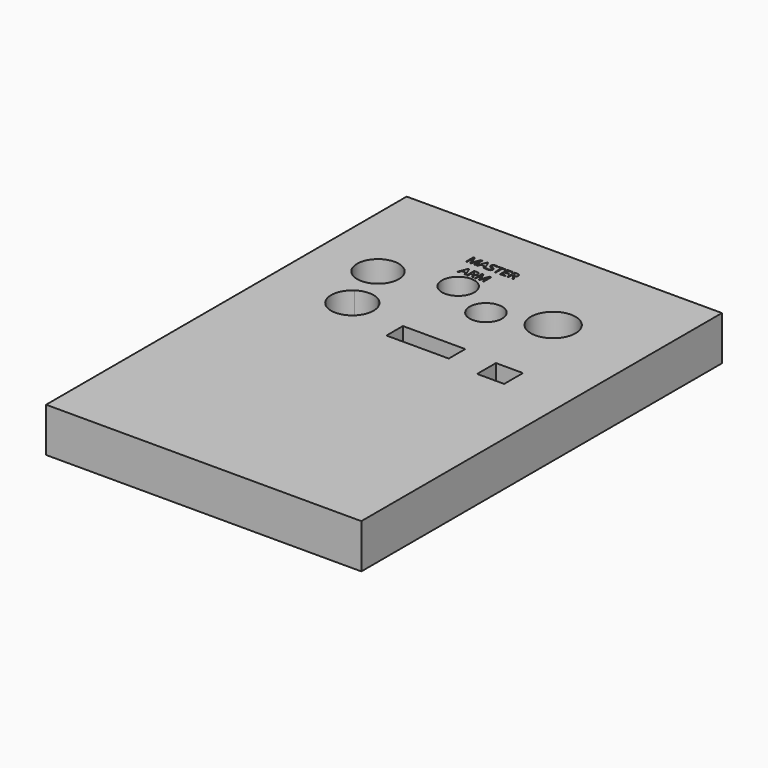
from build123d import *

# Parameters (mm, degrees)
F0_W     = 178
F0_H     = 254.5
F0_R     = 11.7739294938
F0_R_2   = 9.1574293731
F0_W_2   = 35.1873915642
F0_H_2   = 11.6184782237
F0_R_3   = 9.1574274825
F0_W_3   = 15.2700021863
F0_H_3   = 13.2782608271
F0_R_4   = 12.6405317235
F1_DEPTH = 25
F2_DEPTH = 25


with BuildPart() as f1:
    # F0 (on Top) → F1 (new body)
    with BuildSketch(Plane.XY):
        Rectangle(F0_W, F0_H)
        with Locations((-54.2288012803, 63.5412633419)):
            Circle(F0_R, mode=Mode.SUBTRACT)
        with BuildLine():
            ThreePointArc((-32.2966329035, 33.0012664199), (-49.9168302008, 22.4429384628), (-50.9175227463, 42.9599620402))
            ThreePointArc((-50.9175227463, 42.9599620402), (-44.2700982094, 44.9747317258), (-37.6226736725, 42.9599620402))
            ThreePointArc((-37.6226736725, 42.9599620402), (-33.7117702523, 38.6479984113), (-32.2966329035, 33.0012664199))
        make_face(mode=Mode.SUBTRACT)
        Polygon((-22.1080133536, 85.1738999287), (-22.7346302224, 85.1738999287), (-23.3828938556, 86.8293077656), (-25.4689583768, 86.8293077656), (-26.1092468863, 85.1738999287), (-26.7221921143, 85.1738999287), (-24.6646101781, 90.4010239174), (-24.1553415593, 90.4010239174), align=None, mode=Mode.SUBTRACT)
        with Locations((-17.7135802805, 74.4958370924)):
            Circle(F0_R_2, mode=Mode.SUBTRACT)
        with BuildLine():
            Line((-19.7006652743, 87.3385763844), (-20.7875607157, 87.3385763844))
            Line((-20.7875607157, 87.3385763844), (-20.7875607157, 85.1738999287))
            Line((-20.7875607157, 85.1738999287), (-21.3925308199, 85.1738999287))
            Line((-21.3925308199, 85.1738999287), (-21.3925308199, 90.3793771528))
            Line((-21.3925308199, 90.3793771528), (-19.9649836626, 90.3793771528))
            add(Edge.make_bspline(
                [(-19.9649836626, 90.3793771528), (-19.0068295051, 90.3793771528), (-18.5493991909, 90.0125214588)],
                knots=[0, 0, 0, 1, 1, 1], degree=2))
            add(Edge.make_bspline(
                [(-18.5493991909, 90.0125214588), (-18.0919688767, 89.6456657647), (-18.0919688767, 88.9085364664)],
                knots=[0, 0, 0, 1, 1, 1], degree=2))
            add(Edge.make_bspline(
                [(-18.0919688767, 88.9085364664), (-18.0919688767, 87.8763275881), (-19.1389886992, 87.5128898042)],
                knots=[0, 0, 0, 1, 1, 1], degree=2))
            Line((-19.1389886992, 87.5128898042), (-17.7251131827, 85.1738999287))
            Line((-17.7251131827, 85.1738999287), (-18.4405957164, 85.1738999287))
            Line((-18.4405957164, 85.1738999287), (-19.7006652743, 87.3385763844))
        make_face(mode=Mode.SUBTRACT)
        with BuildLine():
            Line((-14.0941532542, 85.1738999287), (-14.5817751084, 85.1738999287))
            Line((-14.5817751084, 85.1738999287), (-16.3476953749, 89.7880786894))
            Line((-16.3476953749, 89.7880786894), (-16.3761779598, 89.7880786894))
            add(Edge.make_bspline(
                [(-16.3761779598, 89.7880786894), (-16.3260486103, 89.2400737551), (-16.3260486103, 88.4847156024)],
                knots=[0, 0, 0, 1, 1, 1], degree=2))
            Line((-16.3260486103, 88.4847156024), (-16.3260486103, 85.1738999287))
            Line((-16.3260486103, 85.1738999287), (-16.8854465786, 85.1738999287))
            Line((-16.8854465786, 85.1738999287), (-16.8854465786, 90.3793771528))
            Line((-16.8854465786, 90.3793771528), (-15.9740038604, 90.3793771528))
            Line((-15.9740038604, 90.3793771528), (-14.3254318439, 86.0853426469))
            Line((-14.3254318439, 86.0853426469), (-14.296949259, 86.0853426469))
            Line((-14.296949259, 86.0853426469), (-12.6347056018, 90.3793771528))
            Line((-12.6347056018, 90.3793771528), (-11.730098704, 90.3793771528))
            Line((-11.730098704, 90.3793771528), (-11.730098704, 85.1738999287))
            Line((-11.730098704, 85.1738999287), (-12.3350688082, 85.1738999287))
            Line((-12.3350688082, 85.1738999287), (-12.3350688082, 88.5280091316))
            add(Edge.make_bspline(
                [(-12.3350688082, 88.5280091316), (-12.3350688082, 89.1044966508), (-12.2849394587, 89.781242869)],
                knots=[0, 0, 0, 1, 1, 1], degree=2))
            Line((-12.2849394587, 89.781242869), (-12.3134220436, 89.781242869))
            Line((-12.3134220436, 89.781242869), (-14.0941532542, 85.1738999287))
        make_face(mode=Mode.SUBTRACT)
        with BuildLine():
            Line((-27.0047393569, 95.0903967023), (-27.4923612111, 95.0903967023))
            Line((-27.4923612111, 95.0903967023), (-29.2582814776, 99.704575463))
            Line((-29.2582814776, 99.704575463), (-29.2867640625, 99.704575463))
            add(Edge.make_bspline(
                [(-29.2867640625, 99.704575463), (-29.236634713, 99.1565705287), (-29.236634713, 98.401212376)],
                knots=[0, 0, 0, 1, 1, 1], degree=2))
            Line((-29.236634713, 98.401212376), (-29.236634713, 95.0903967023))
            Line((-29.236634713, 95.0903967023), (-29.7960326813, 95.0903967023))
            Line((-29.7960326813, 95.0903967023), (-29.7960326813, 100.2958739264))
            Line((-29.7960326813, 100.2958739264), (-28.8845899631, 100.2958739264))
            Line((-28.8845899631, 100.2958739264), (-27.2360179467, 96.0018394204))
            Line((-27.2360179467, 96.0018394204), (-27.2075353617, 96.0018394204))
            Line((-27.2075353617, 96.0018394204), (-25.5452917045, 100.2958739264))
            Line((-25.5452917045, 100.2958739264), (-24.6406848067, 100.2958739264))
            Line((-24.6406848067, 100.2958739264), (-24.6406848067, 95.0903967023))
            Line((-24.6406848067, 95.0903967023), (-25.2456549109, 95.0903967023))
            Line((-25.2456549109, 95.0903967023), (-25.2456549109, 98.4445059051))
            add(Edge.make_bspline(
                [(-25.2456549109, 98.4445059051), (-25.2456549109, 99.0209934243), (-25.1955255614, 99.6977396426)],
                knots=[0, 0, 0, 1, 1, 1], degree=2))
            Line((-25.1955255614, 99.6977396426), (-25.2240081463, 99.6977396426))
            Line((-25.2240081463, 99.6977396426), (-27.0047393569, 95.0903967023))
        make_face(mode=Mode.SUBTRACT)
        Polygon((-19.3144414225, 95.0903967023), (-19.9410582912, 95.0903967023), (-20.5893219245, 96.7458045391), (-22.6753864457, 96.7458045391), (-23.3156749552, 95.0903967023), (-23.9286201831, 95.0903967023), (-21.8710382469, 100.3175206909), (-21.3617696281, 100.3175206909), align=None, mode=Mode.SUBTRACT)
        with BuildLine():
            add(Edge.make_bspline(
                [(-15.9694466468, 97.3439388229), (-15.6618347294, 97.008983624), (-15.6618347294, 96.4757896339)],
                knots=[0, 0, 0, 1, 1, 1], degree=2))
            add(Edge.make_bspline(
                [(-15.6618347294, 96.4757896339), (-15.6618347294, 95.7887896851), (-16.1602799659, 95.4037051367)],
                knots=[0, 0, 0, 1, 1, 1], degree=2))
            add(Edge.make_bspline(
                [(-16.1602799659, 95.4037051367), (-16.6587252024, 95.0186205882), (-17.5132027507, 95.0186205882)],
                knots=[0, 0, 0, 1, 1, 1], degree=2))
            add(Edge.make_bspline(
                [(-17.5132027507, 95.0186205882), (-18.4383171096, 95.0186205882), (-18.9373319978, 95.2578743018)],
                knots=[0, 0, 0, 1, 1, 1], degree=2))
            Line((-18.9373319978, 95.2578743018), (-18.9373319978, 95.8411976414))
            add(Edge.make_bspline(
                [(-18.9373319978, 95.8411976414), (-18.6160484397, 95.7067598404), (-18.238939015, 95.628147906)],
                knots=[0, 0, 0, 1, 1, 1], degree=2))
            add(Edge.make_bspline(
                [(-18.238939015, 95.628147906), (-17.8618295904, 95.5495359716), (-17.4915559861, 95.5495359716)],
                knots=[0, 0, 0, 1, 1, 1], degree=2))
            add(Edge.make_bspline(
                [(-17.4915559861, 95.5495359716), (-16.886585882, 95.5495359716), (-16.580113268, 95.7791056062)],
                knots=[0, 0, 0, 1, 1, 1], degree=2))
            add(Edge.make_bspline(
                [(-16.580113268, 95.7791056062), (-16.273640654, 96.0086752408), (-16.273640654, 96.418824464)],
                knots=[0, 0, 0, 1, 1, 1], degree=2))
            add(Edge.make_bspline(
                [(-16.273640654, 96.418824464), (-16.273640654, 96.6888393693), (-16.3824441285, 96.861443834)],
                knots=[0, 0, 0, 1, 1, 1], degree=2))
            add(Edge.make_bspline(
                [(-16.3824441285, 96.861443834), (-16.491247603, 97.0340482988), (-16.7458819124, 97.1804487854)],
                knots=[0, 0, 0, 1, 1, 1], degree=2))
            add(Edge.make_bspline(
                [(-16.7458819124, 97.1804487854), (-17.0005162217, 97.326849272), (-17.5200385711, 97.5114164224)],
                knots=[0, 0, 0, 1, 1, 1], degree=2))
            add(Edge.make_bspline(
                [(-17.5200385711, 97.5114164224), (-18.2457748354, 97.7711775971), (-18.5573743147, 98.1272099089)],
                knots=[0, 0, 0, 1, 1, 1], degree=2))
            add(Edge.make_bspline(
                [(-18.5573743147, 98.1272099089), (-18.868973794, 98.4832422206), (-18.868973794, 99.0563118297)],
                knots=[0, 0, 0, 1, 1, 1], degree=2))
            add(Edge.make_bspline(
                [(-18.868973794, 99.0563118297), (-18.868973794, 99.6578640237), (-18.4172399968, 100.0138963354)],
                knots=[0, 0, 0, 1, 1, 1], degree=2))
            add(Edge.make_bspline(
                [(-18.4172399968, 100.0138963354), (-17.9655061996, 100.3699286472), (-17.2204017775, 100.3699286472)],
                knots=[0, 0, 0, 1, 1, 1], degree=2))
            add(Edge.make_bspline(
                [(-17.2204017775, 100.3699286472), (-16.4445361637, 100.3699286472), (-15.7928546202, 100.0851027978)],
                knots=[0, 0, 0, 1, 1, 1], degree=2))
            Line((-15.7928546202, 100.0851027978), (-15.9819789842, 99.5587446281))
            add(Edge.make_bspline(
                [(-15.9819789842, 99.5587446281), (-16.6268247073, 99.8287595333), (-17.2352127217, 99.8287595333)],
                knots=[0, 0, 0, 1, 1, 1], degree=2))
            add(Edge.make_bspline(
                [(-17.2352127217, 99.8287595333), (-17.7159987555, 99.8287595333), (-17.9865833124, 99.6225456183)],
                knots=[0, 0, 0, 1, 1, 1], degree=2))
            add(Edge.make_bspline(
                [(-17.9865833124, 99.6225456183), (-18.2571678694, 99.4163317033), (-18.2571678694, 99.0494760093)],
                knots=[0, 0, 0, 1, 1, 1], degree=2))
            add(Edge.make_bspline(
                [(-18.2571678694, 99.0494760093), (-18.2571678694, 98.779461104), (-18.1574788221, 98.6062869876)],
                knots=[0, 0, 0, 1, 1, 1], degree=2))
            add(Edge.make_bspline(
                [(-18.1574788221, 98.6062869876), (-18.0577897748, 98.4331128711), (-17.8208146681, 98.2889909913)],
                knots=[0, 0, 0, 1, 1, 1], degree=2))
            add(Edge.make_bspline(
                [(-17.8208146681, 98.2889909913), (-17.5838395614, 98.1448691115), (-17.0962177071, 97.9705556917)],
                knots=[0, 0, 0, 1, 1, 1], degree=2))
            add(Edge.make_bspline(
                [(-17.0962177071, 97.9705556917), (-16.2770585642, 97.6788940219), (-15.9694466468, 97.3439388229)],
                knots=[0, 0, 0, 1, 1, 1], degree=2))
        make_face(mode=Mode.SUBTRACT)
        Polygon((-12.9947254754, 99.7581227227), (-12.9947254754, 95.0903967023), (-13.5996955796, 95.0903967023), (-13.5996955796, 99.7581227227), (-15.2482675961, 99.7581227227), (-15.2482675961, 100.2958739264), (-11.346153459, 100.2958739264), (-11.346153459, 99.7581227227), align=None, mode=Mode.SUBTRACT)
        Polygon((-7.6605069674, 95.6315658162), (-7.6605069674, 95.0903967023), (-10.5623127214, 95.0903967023), (-10.5623127214, 100.2958739264), (-7.6605069674, 100.2958739264), (-7.6605069674, 99.7581227227), (-9.9573426172, 99.7581227227), (-9.9573426172, 98.0810681212), (-7.7995019819, 98.0810681212), (-7.7995019819, 97.5467348277), (-9.9573426172, 97.5467348277), (-9.9573426172, 95.6315658162), align=None, mode=Mode.SUBTRACT)
        with BuildLine():
            Line((-4.8156663834, 97.2550731579), (-5.9025618248, 97.2550731579))
            Line((-5.9025618248, 97.2550731579), (-5.9025618248, 95.0903967023))
            Line((-5.9025618248, 95.0903967023), (-6.5075319289, 95.0903967023))
            Line((-6.5075319289, 95.0903967023), (-6.5075319289, 100.2958739264))
            Line((-6.5075319289, 100.2958739264), (-5.0799847716, 100.2958739264))
            add(Edge.make_bspline(
                [(-5.0799847716, 100.2958739264), (-4.1218306142, 100.2958739264), (-3.6644003, 99.9290182323)],
                knots=[0, 0, 0, 1, 1, 1], degree=2))
            add(Edge.make_bspline(
                [(-3.6644003, 99.9290182323), (-3.2069699858, 99.5621625383), (-3.2069699858, 98.8250332399)],
                knots=[0, 0, 0, 1, 1, 1], degree=2))
            add(Edge.make_bspline(
                [(-3.2069699858, 98.8250332399), (-3.2069699858, 97.7928243616), (-4.2539898083, 97.4293865778)],
                knots=[0, 0, 0, 1, 1, 1], degree=2))
            Line((-4.2539898083, 97.4293865778), (-2.8401142918, 95.0903967023))
            Line((-2.8401142918, 95.0903967023), (-3.5555968255, 95.0903967023))
            Line((-3.5555968255, 95.0903967023), (-4.8156663834, 97.2550731579))
        make_face(mode=Mode.SUBTRACT)
        with Locations((4.5275064185, 23.8724621013)):
            Rectangle(F0_W_2, F0_H_2, mode=Mode.SUBTRACT)
        with Locations((7.5151156634, 62.5453963876)):
            Circle(F0_R_3, mode=Mode.SUBTRACT)
        with Locations((48.6777238548, 21.050831303)):
            Rectangle(F0_W_3, F0_H_3, mode=Mode.SUBTRACT)
        with Locations((38.0551144481, 71.8401819468)):
            Circle(F0_R_4, mode=Mode.SUBTRACT)
    extrude(amount=F1_DEPTH)

    # F0 (on Top) → F2 (cut)
    with BuildSketch(Plane.XY):
        Rectangle(F0_W, F0_H)
        with Locations((-54.2288012803, 63.5412633419)):
            Circle(F0_R, mode=Mode.SUBTRACT)
        with BuildLine():
            ThreePointArc((-32.2966329035, 33.0012664199), (-49.9168302008, 22.4429384628), (-50.9175227463, 42.9599620402))
            ThreePointArc((-50.9175227463, 42.9599620402), (-44.2700982094, 44.9747317258), (-37.6226736725, 42.9599620402))
            ThreePointArc((-37.6226736725, 42.9599620402), (-33.7117702523, 38.6479984113), (-32.2966329035, 33.0012664199))
        make_face(mode=Mode.SUBTRACT)
        Polygon((-22.1080133536, 85.1738999287), (-22.7346302224, 85.1738999287), (-23.3828938556, 86.8293077656), (-25.4689583768, 86.8293077656), (-26.1092468863, 85.1738999287), (-26.7221921143, 85.1738999287), (-24.6646101781, 90.4010239174), (-24.1553415593, 90.4010239174), align=None, mode=Mode.SUBTRACT)
        with Locations((-17.7135802805, 74.4958370924)):
            Circle(F0_R_2, mode=Mode.SUBTRACT)
        with BuildLine():
            Line((-19.7006652743, 87.3385763844), (-20.7875607157, 87.3385763844))
            Line((-20.7875607157, 87.3385763844), (-20.7875607157, 85.1738999287))
            Line((-20.7875607157, 85.1738999287), (-21.3925308199, 85.1738999287))
            Line((-21.3925308199, 85.1738999287), (-21.3925308199, 90.3793771528))
            Line((-21.3925308199, 90.3793771528), (-19.9649836626, 90.3793771528))
            add(Edge.make_bspline(
                [(-19.9649836626, 90.3793771528), (-19.0068295051, 90.3793771528), (-18.5493991909, 90.0125214588)],
                knots=[0, 0, 0, 1, 1, 1], degree=2))
            add(Edge.make_bspline(
                [(-18.5493991909, 90.0125214588), (-18.0919688767, 89.6456657647), (-18.0919688767, 88.9085364664)],
                knots=[0, 0, 0, 1, 1, 1], degree=2))
            add(Edge.make_bspline(
                [(-18.0919688767, 88.9085364664), (-18.0919688767, 87.8763275881), (-19.1389886992, 87.5128898042)],
                knots=[0, 0, 0, 1, 1, 1], degree=2))
            Line((-19.1389886992, 87.5128898042), (-17.7251131827, 85.1738999287))
            Line((-17.7251131827, 85.1738999287), (-18.4405957164, 85.1738999287))
            Line((-18.4405957164, 85.1738999287), (-19.7006652743, 87.3385763844))
        make_face(mode=Mode.SUBTRACT)
        with BuildLine():
            Line((-14.0941532542, 85.1738999287), (-14.5817751084, 85.1738999287))
            Line((-14.5817751084, 85.1738999287), (-16.3476953749, 89.7880786894))
            Line((-16.3476953749, 89.7880786894), (-16.3761779598, 89.7880786894))
            add(Edge.make_bspline(
                [(-16.3761779598, 89.7880786894), (-16.3260486103, 89.2400737551), (-16.3260486103, 88.4847156024)],
                knots=[0, 0, 0, 1, 1, 1], degree=2))
            Line((-16.3260486103, 88.4847156024), (-16.3260486103, 85.1738999287))
            Line((-16.3260486103, 85.1738999287), (-16.8854465786, 85.1738999287))
            Line((-16.8854465786, 85.1738999287), (-16.8854465786, 90.3793771528))
            Line((-16.8854465786, 90.3793771528), (-15.9740038604, 90.3793771528))
            Line((-15.9740038604, 90.3793771528), (-14.3254318439, 86.0853426469))
            Line((-14.3254318439, 86.0853426469), (-14.296949259, 86.0853426469))
            Line((-14.296949259, 86.0853426469), (-12.6347056018, 90.3793771528))
            Line((-12.6347056018, 90.3793771528), (-11.730098704, 90.3793771528))
            Line((-11.730098704, 90.3793771528), (-11.730098704, 85.1738999287))
            Line((-11.730098704, 85.1738999287), (-12.3350688082, 85.1738999287))
            Line((-12.3350688082, 85.1738999287), (-12.3350688082, 88.5280091316))
            add(Edge.make_bspline(
                [(-12.3350688082, 88.5280091316), (-12.3350688082, 89.1044966508), (-12.2849394587, 89.781242869)],
                knots=[0, 0, 0, 1, 1, 1], degree=2))
            Line((-12.2849394587, 89.781242869), (-12.3134220436, 89.781242869))
            Line((-12.3134220436, 89.781242869), (-14.0941532542, 85.1738999287))
        make_face(mode=Mode.SUBTRACT)
        with BuildLine():
            Line((-27.0047393569, 95.0903967023), (-27.4923612111, 95.0903967023))
            Line((-27.4923612111, 95.0903967023), (-29.2582814776, 99.704575463))
            Line((-29.2582814776, 99.704575463), (-29.2867640625, 99.704575463))
            add(Edge.make_bspline(
                [(-29.2867640625, 99.704575463), (-29.236634713, 99.1565705287), (-29.236634713, 98.401212376)],
                knots=[0, 0, 0, 1, 1, 1], degree=2))
            Line((-29.236634713, 98.401212376), (-29.236634713, 95.0903967023))
            Line((-29.236634713, 95.0903967023), (-29.7960326813, 95.0903967023))
            Line((-29.7960326813, 95.0903967023), (-29.7960326813, 100.2958739264))
            Line((-29.7960326813, 100.2958739264), (-28.8845899631, 100.2958739264))
            Line((-28.8845899631, 100.2958739264), (-27.2360179467, 96.0018394204))
            Line((-27.2360179467, 96.0018394204), (-27.2075353617, 96.0018394204))
            Line((-27.2075353617, 96.0018394204), (-25.5452917045, 100.2958739264))
            Line((-25.5452917045, 100.2958739264), (-24.6406848067, 100.2958739264))
            Line((-24.6406848067, 100.2958739264), (-24.6406848067, 95.0903967023))
            Line((-24.6406848067, 95.0903967023), (-25.2456549109, 95.0903967023))
            Line((-25.2456549109, 95.0903967023), (-25.2456549109, 98.4445059051))
            add(Edge.make_bspline(
                [(-25.2456549109, 98.4445059051), (-25.2456549109, 99.0209934243), (-25.1955255614, 99.6977396426)],
                knots=[0, 0, 0, 1, 1, 1], degree=2))
            Line((-25.1955255614, 99.6977396426), (-25.2240081463, 99.6977396426))
            Line((-25.2240081463, 99.6977396426), (-27.0047393569, 95.0903967023))
        make_face(mode=Mode.SUBTRACT)
        Polygon((-19.3144414225, 95.0903967023), (-19.9410582912, 95.0903967023), (-20.5893219245, 96.7458045391), (-22.6753864457, 96.7458045391), (-23.3156749552, 95.0903967023), (-23.9286201831, 95.0903967023), (-21.8710382469, 100.3175206909), (-21.3617696281, 100.3175206909), align=None, mode=Mode.SUBTRACT)
        with BuildLine():
            add(Edge.make_bspline(
                [(-15.9694466468, 97.3439388229), (-15.6618347294, 97.008983624), (-15.6618347294, 96.4757896339)],
                knots=[0, 0, 0, 1, 1, 1], degree=2))
            add(Edge.make_bspline(
                [(-15.6618347294, 96.4757896339), (-15.6618347294, 95.7887896851), (-16.1602799659, 95.4037051367)],
                knots=[0, 0, 0, 1, 1, 1], degree=2))
            add(Edge.make_bspline(
                [(-16.1602799659, 95.4037051367), (-16.6587252024, 95.0186205882), (-17.5132027507, 95.0186205882)],
                knots=[0, 0, 0, 1, 1, 1], degree=2))
            add(Edge.make_bspline(
                [(-17.5132027507, 95.0186205882), (-18.4383171096, 95.0186205882), (-18.9373319978, 95.2578743018)],
                knots=[0, 0, 0, 1, 1, 1], degree=2))
            Line((-18.9373319978, 95.2578743018), (-18.9373319978, 95.8411976414))
            add(Edge.make_bspline(
                [(-18.9373319978, 95.8411976414), (-18.6160484397, 95.7067598404), (-18.238939015, 95.628147906)],
                knots=[0, 0, 0, 1, 1, 1], degree=2))
            add(Edge.make_bspline(
                [(-18.238939015, 95.628147906), (-17.8618295904, 95.5495359716), (-17.4915559861, 95.5495359716)],
                knots=[0, 0, 0, 1, 1, 1], degree=2))
            add(Edge.make_bspline(
                [(-17.4915559861, 95.5495359716), (-16.886585882, 95.5495359716), (-16.580113268, 95.7791056062)],
                knots=[0, 0, 0, 1, 1, 1], degree=2))
            add(Edge.make_bspline(
                [(-16.580113268, 95.7791056062), (-16.273640654, 96.0086752408), (-16.273640654, 96.418824464)],
                knots=[0, 0, 0, 1, 1, 1], degree=2))
            add(Edge.make_bspline(
                [(-16.273640654, 96.418824464), (-16.273640654, 96.6888393693), (-16.3824441285, 96.861443834)],
                knots=[0, 0, 0, 1, 1, 1], degree=2))
            add(Edge.make_bspline(
                [(-16.3824441285, 96.861443834), (-16.491247603, 97.0340482988), (-16.7458819124, 97.1804487854)],
                knots=[0, 0, 0, 1, 1, 1], degree=2))
            add(Edge.make_bspline(
                [(-16.7458819124, 97.1804487854), (-17.0005162217, 97.326849272), (-17.5200385711, 97.5114164224)],
                knots=[0, 0, 0, 1, 1, 1], degree=2))
            add(Edge.make_bspline(
                [(-17.5200385711, 97.5114164224), (-18.2457748354, 97.7711775971), (-18.5573743147, 98.1272099089)],
                knots=[0, 0, 0, 1, 1, 1], degree=2))
            add(Edge.make_bspline(
                [(-18.5573743147, 98.1272099089), (-18.868973794, 98.4832422206), (-18.868973794, 99.0563118297)],
                knots=[0, 0, 0, 1, 1, 1], degree=2))
            add(Edge.make_bspline(
                [(-18.868973794, 99.0563118297), (-18.868973794, 99.6578640237), (-18.4172399968, 100.0138963354)],
                knots=[0, 0, 0, 1, 1, 1], degree=2))
            add(Edge.make_bspline(
                [(-18.4172399968, 100.0138963354), (-17.9655061996, 100.3699286472), (-17.2204017775, 100.3699286472)],
                knots=[0, 0, 0, 1, 1, 1], degree=2))
            add(Edge.make_bspline(
                [(-17.2204017775, 100.3699286472), (-16.4445361637, 100.3699286472), (-15.7928546202, 100.0851027978)],
                knots=[0, 0, 0, 1, 1, 1], degree=2))
            Line((-15.7928546202, 100.0851027978), (-15.9819789842, 99.5587446281))
            add(Edge.make_bspline(
                [(-15.9819789842, 99.5587446281), (-16.6268247073, 99.8287595333), (-17.2352127217, 99.8287595333)],
                knots=[0, 0, 0, 1, 1, 1], degree=2))
            add(Edge.make_bspline(
                [(-17.2352127217, 99.8287595333), (-17.7159987555, 99.8287595333), (-17.9865833124, 99.6225456183)],
                knots=[0, 0, 0, 1, 1, 1], degree=2))
            add(Edge.make_bspline(
                [(-17.9865833124, 99.6225456183), (-18.2571678694, 99.4163317033), (-18.2571678694, 99.0494760093)],
                knots=[0, 0, 0, 1, 1, 1], degree=2))
            add(Edge.make_bspline(
                [(-18.2571678694, 99.0494760093), (-18.2571678694, 98.779461104), (-18.1574788221, 98.6062869876)],
                knots=[0, 0, 0, 1, 1, 1], degree=2))
            add(Edge.make_bspline(
                [(-18.1574788221, 98.6062869876), (-18.0577897748, 98.4331128711), (-17.8208146681, 98.2889909913)],
                knots=[0, 0, 0, 1, 1, 1], degree=2))
            add(Edge.make_bspline(
                [(-17.8208146681, 98.2889909913), (-17.5838395614, 98.1448691115), (-17.0962177071, 97.9705556917)],
                knots=[0, 0, 0, 1, 1, 1], degree=2))
            add(Edge.make_bspline(
                [(-17.0962177071, 97.9705556917), (-16.2770585642, 97.6788940219), (-15.9694466468, 97.3439388229)],
                knots=[0, 0, 0, 1, 1, 1], degree=2))
        make_face(mode=Mode.SUBTRACT)
        Polygon((-12.9947254754, 99.7581227227), (-12.9947254754, 95.0903967023), (-13.5996955796, 95.0903967023), (-13.5996955796, 99.7581227227), (-15.2482675961, 99.7581227227), (-15.2482675961, 100.2958739264), (-11.346153459, 100.2958739264), (-11.346153459, 99.7581227227), align=None, mode=Mode.SUBTRACT)
        Polygon((-7.6605069674, 95.6315658162), (-7.6605069674, 95.0903967023), (-10.5623127214, 95.0903967023), (-10.5623127214, 100.2958739264), (-7.6605069674, 100.2958739264), (-7.6605069674, 99.7581227227), (-9.9573426172, 99.7581227227), (-9.9573426172, 98.0810681212), (-7.7995019819, 98.0810681212), (-7.7995019819, 97.5467348277), (-9.9573426172, 97.5467348277), (-9.9573426172, 95.6315658162), align=None, mode=Mode.SUBTRACT)
        with BuildLine():
            Line((-4.8156663834, 97.2550731579), (-5.9025618248, 97.2550731579))
            Line((-5.9025618248, 97.2550731579), (-5.9025618248, 95.0903967023))
            Line((-5.9025618248, 95.0903967023), (-6.5075319289, 95.0903967023))
            Line((-6.5075319289, 95.0903967023), (-6.5075319289, 100.2958739264))
            Line((-6.5075319289, 100.2958739264), (-5.0799847716, 100.2958739264))
            add(Edge.make_bspline(
                [(-5.0799847716, 100.2958739264), (-4.1218306142, 100.2958739264), (-3.6644003, 99.9290182323)],
                knots=[0, 0, 0, 1, 1, 1], degree=2))
            add(Edge.make_bspline(
                [(-3.6644003, 99.9290182323), (-3.2069699858, 99.5621625383), (-3.2069699858, 98.8250332399)],
                knots=[0, 0, 0, 1, 1, 1], degree=2))
            add(Edge.make_bspline(
                [(-3.2069699858, 98.8250332399), (-3.2069699858, 97.7928243616), (-4.2539898083, 97.4293865778)],
                knots=[0, 0, 0, 1, 1, 1], degree=2))
            Line((-4.2539898083, 97.4293865778), (-2.8401142918, 95.0903967023))
            Line((-2.8401142918, 95.0903967023), (-3.5555968255, 95.0903967023))
            Line((-3.5555968255, 95.0903967023), (-4.8156663834, 97.2550731579))
        make_face(mode=Mode.SUBTRACT)
        with Locations((4.5275064185, 23.8724621013)):
            Rectangle(F0_W_2, F0_H_2, mode=Mode.SUBTRACT)
        with Locations((7.5151156634, 62.5453963876)):
            Circle(F0_R_3, mode=Mode.SUBTRACT)
        with Locations((48.6777238548, 21.050831303)):
            Rectangle(F0_W_3, F0_H_3, mode=Mode.SUBTRACT)
        with Locations((38.0551144481, 71.8401819468)):
            Circle(F0_R_4, mode=Mode.SUBTRACT)
    extrude(amount=-F2_DEPTH, mode=Mode.SUBTRACT)


solid = f1.part
